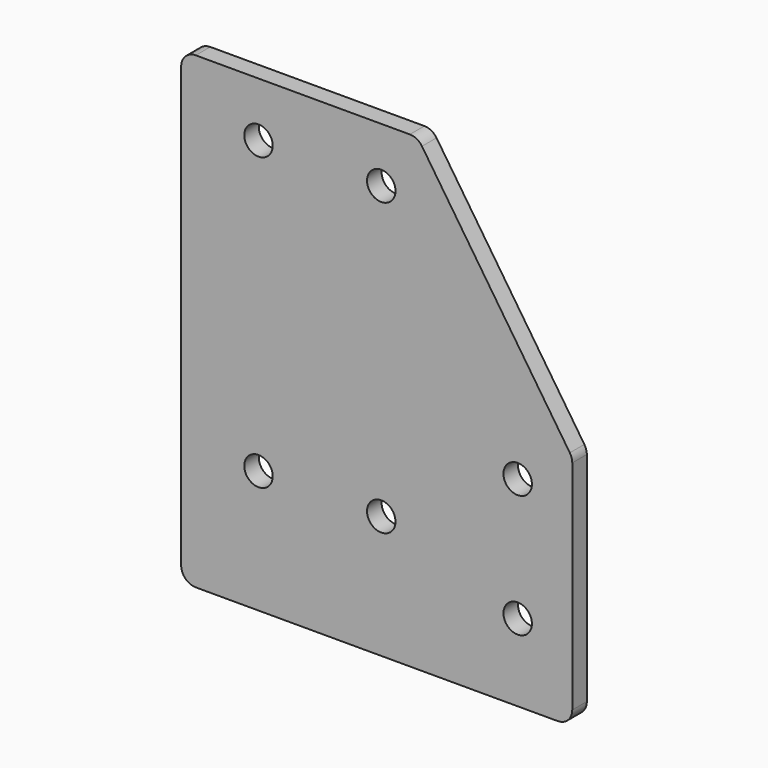
from build123d import *

# Parameters (mm, degrees)
F0_R     = 4.9657
F1_DEPTH = 6.35
F2_R     = 5.08


# Not quite as in the source:
# - a feature names something its author has since deleted; it is built from what else it names


with BuildPart() as f1:
    # F0 (on Front) → F1 (new body)
    with BuildSketch(Plane.XZ):
        Polygon((-120.1667662859, -0.1937935591), (16.3582337141, -0.1937935591), (16.3582337141, 82.3562064409), (-37.6167662859, 163.3187064409), (-120.1667662859, 163.3187064409), (-120.1667662859, 144.2687064409), align=None)
        with Locations((-93.1792662859, 42.6687064409)):
            Circle(F0_R, mode=Mode.SUBTRACT)
        with Locations((-50.3167662859, 42.6687064409)):
            Circle(F0_R, mode=Mode.SUBTRACT)
        with Locations((-2.6917662859, 26.7937064409)):
            Circle(F0_R, mode=Mode.SUBTRACT)
        with Locations((-2.6917662859, 69.6562064409)):
            Circle(F0_R, mode=Mode.SUBTRACT)
        with BuildLine():
            ThreePointArc((-88.2135662859, 144.2687064409), (-93.1792662859, 139.3030064409), (-98.1449662859, 144.2687064409))
            ThreePointArc((-98.1449662859, 144.2687064409), (-93.1792662859, 149.2344064409), (-88.2135662859, 144.2687064409))
        make_face(mode=Mode.SUBTRACT)
        with Locations((-50.3167662859, 144.2687064409)):
            Circle(F0_R, mode=Mode.SUBTRACT)
    extrude(amount=F1_DEPTH)

    # F2
    f2_edges = [f1.edges().sort_by_distance(p)[0] for p in [
        (-37.616766, -3.175, 163.318706),
        (16.358234, -3.175, 82.356206),
        (16.358234, -3.175, -0.193794),
        (-120.166766, -3.175, -0.193794),
        (-120.166766, -3.175, 163.318706),
    ]]
    fillet(f2_edges, radius=F2_R)


solid = f1.part
